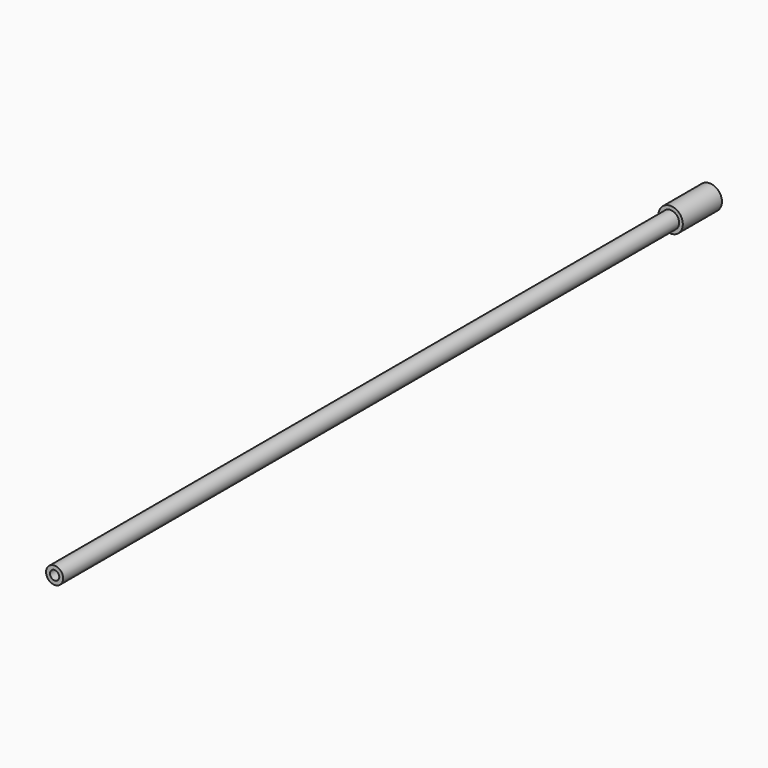
from build123d import *

# Parameters (mm, degrees)
F0_R     = 7
F0_R_2   = 3.81
F1_DEPTH = 630
F2_R     = 10
F2_R_2   = 7
F2_R_3   = 3.81
F3_DEPTH = 40
F4_W     = 4.28
F4_H     = 4.36


with BuildPart() as f1:
    # F0 (on Front) → F1 (new body)
    with BuildSketch(Plane.XZ):
        Circle(F0_R)
        Circle(F0_R_2, mode=Mode.SUBTRACT)
    extrude(amount=F1_DEPTH)

    # F2 (on face) → F3 (join)
    with BuildSketch(Plane(origin=(0, 0, 0), x_dir=(-1, 0, 0), z_dir=(0, 1, 0))):
        Circle(F2_R)
        Circle(F2_R_2, mode=Mode.SUBTRACT)
        Circle(F2_R_2)
        Circle(F2_R_3, mode=Mode.SUBTRACT)
    extrude(amount=F3_DEPTH)

    # F4 (on Right) → F5 (revolve, cut)
    with BuildSketch(Plane.YZ):
        with Locations((2.14, 2.18)):
            Rectangle(F4_W, F4_H)
        Polygon((4.28, 4.36), (4.28, 0), (11.98, 0), (11.98, 5.765), align=None)
        Polygon((11.98, 5.765), (11.98, 0), (47.75, 0), (47.75, 5.98), align=None)
    revolve(axis=Axis((0, 29.865, 0), (0, 1, 0)), mode=Mode.SUBTRACT)


solid = f1.part
